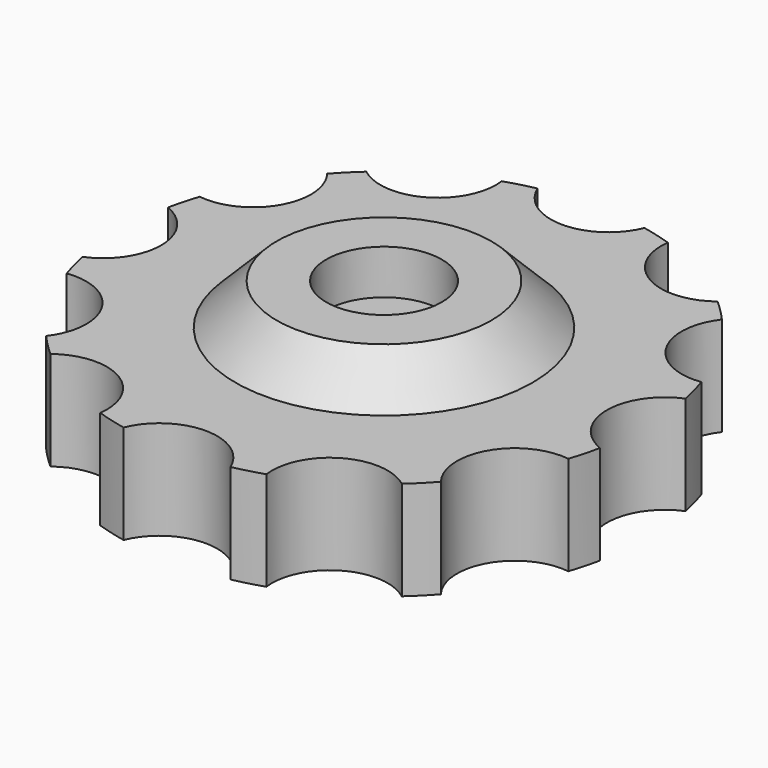
from build123d import *

# Parameters (mm, degrees)
F1_DEPTH = 3
F2_DEPTH = 2.5
F3_R     = 4.5
F4_DEPTH = 1.25
F6_SIZE  = 1.24999
F5_R     = 1.75
F7_DEPTH = 1.35


# Not quite as in the source:
# - a fillet or chamfer is up to 0.001 mm smaller than in the source, because OpenCascade refuses the exact size


with BuildPart() as f1:
    # F0 (on Top) → F1 (new body)
    with BuildSketch(Plane.XY):
        with BuildLine():
            ThreePointArc((7.8345588235, -1.6185450382), (6.75, 0), (7.8345588235, 1.6185450382))
            ThreePointArc((7.8345588235, 1.6185450382), (7.7274066103, 2.0705523608), (7.5941994877, 2.5155782915))
            ThreePointArc((7.5941994877, 2.5155782915), (5.8456714755, 3.375), (5.9756544495, 5.318980532))
            ThreePointArc((5.9756544495, 5.318980532), (5.6568542495, 5.6568542495), (5.318980532, 5.9756544495))
            ThreePointArc((5.318980532, 5.9756544495), (3.375, 5.8456714755), (2.5155782915, 7.5941994877))
            ThreePointArc((2.5155782915, 7.5941994877), (2.0705523608, 7.7274066103), (1.6185450382, 7.8345588235))
            ThreePointArc((1.6185450382, 7.8345588235), (0, 6.75), (-1.6185450382, 7.8345588235))
            ThreePointArc((-1.6185450382, 7.8345588235), (-2.0705523608, 7.7274066103), (-2.5155782915, 7.5941994877))
            ThreePointArc((-2.5155782915, 7.5941994877), (-2.5038989162, 7.4779678276), (-2.5, 7.3612159322))
            ThreePointArc((-2.5, 7.3612159322), (-3.4780595655, 5.7906720883), (-5.318980532, 5.9756544495))
            ThreePointArc((-5.318980532, 5.9756544495), (-5.6568542495, 5.6568542495), (-5.9756544495, 5.318980532))
            ThreePointArc((-5.9756544495, 5.318980532), (-5.7048294141, 4.8146978862), (-5.6112159322, 4.25))
            ThreePointArc((-5.6112159322, 4.25), (-6.2090920721, 2.932764026), (-7.5941994877, 2.5155782915))
            ThreePointArc((-7.5941994877, 2.5155782915), (-7.7274066103, 2.0705523608), (-7.8345588235, 1.6185450382))
            ThreePointArc((-7.8345588235, 1.6185450382), (-7.0462080515, 0.9741606493), (-6.75, 0))
            ThreePointArc((-6.75, 0), (-7.0462080515, -0.9741606493), (-7.8345588235, -1.6185450382))
            ThreePointArc((-7.8345588235, -1.6185450382), (-7.7274066103, -2.0705523608), (-7.5941994877, -2.5155782915))
            ThreePointArc((-7.5941994877, -2.5155782915), (-6.2090920721, -2.932764026), (-5.6112159322, -4.25))
            ThreePointArc((-5.6112159322, -4.25), (-5.7048294141, -4.8146978862), (-5.9756544495, -5.318980532))
            ThreePointArc((-5.9756544495, -5.318980532), (-5.6568542495, -5.6568542495), (-5.318980532, -5.9756544495))
            ThreePointArc((-5.318980532, -5.9756544495), (-3.4780595655, -5.7906720883), (-2.5, -7.3612159322))
            ThreePointArc((-2.5, -7.3612159322), (-2.5038989162, -7.4779678276), (-2.5155782915, -7.5941994877))
            ThreePointArc((-2.5155782915, -7.5941994877), (-2.0705523608, -7.7274066103), (-1.6185450382, -7.8345588235))
            ThreePointArc((-1.6185450382, -7.8345588235), (0, -6.75), (1.6185450382, -7.8345588235))
            ThreePointArc((1.6185450382, -7.8345588235), (2.0705523608, -7.7274066103), (2.5155782915, -7.5941994877))
            ThreePointArc((2.5155782915, -7.5941994877), (3.375, -5.8456714755), (5.318980532, -5.9756544495))
            ThreePointArc((5.318980532, -5.9756544495), (5.6568542495, -5.6568542495), (5.9756544495, -5.318980532))
            ThreePointArc((5.9756544495, -5.318980532), (5.8456714755, -3.375), (7.5941994877, -2.5155782915))
            ThreePointArc((7.5941994877, -2.5155782915), (7.7274066103, -2.0705523608), (7.8345588235, -1.6185450382))
        make_face()
        Polygon((3.4641016151, 0), (1.7320508076, -3), (-1.7320508076, -3), (-3.4641016151, 0), (-1.7320508076, 3), (1.7320508076, 3), align=None, mode=Mode.SUBTRACT)
        Polygon((-1.7320508076, -3), (1.7320508076, -3), (3.4641016151, 0), (1.7320508076, 3), (-1.7320508076, 3), (-3.4641016151, 0), align=None)
    extrude(amount=F1_DEPTH)

    # F0 (on Top) → F2 (cut)
    with BuildSketch(Plane.XY):
        Polygon((-1.7320508076, -3), (1.7320508076, -3), (3.4641016151, 0), (1.7320508076, 3), (-1.7320508076, 3), (-3.4641016151, 0), align=None)
    extrude(amount=F2_DEPTH, mode=Mode.SUBTRACT)

    # F3 (on face) → F4 (join)
    with BuildSketch(Plane.XY.offset(3)):
        Circle(F3_R)
    extrude(amount=F4_DEPTH)

    # F6 (size 1.25 in the source; OpenCascade refuses exactly that, so slightly less here)
    f6_edges = [f1.edges().sort_by_distance(p)[0] for p in [
        (-4.5, 0, 4.25),
    ]]
    chamfer(f6_edges, length=F6_SIZE)

    # F5 (on face) → F7 (cut)
    with BuildSketch(Plane.XY.offset(4.25)):
        Circle(F5_R)
    extrude(amount=-F7_DEPTH, mode=Mode.SUBTRACT)


solid = f1.part
